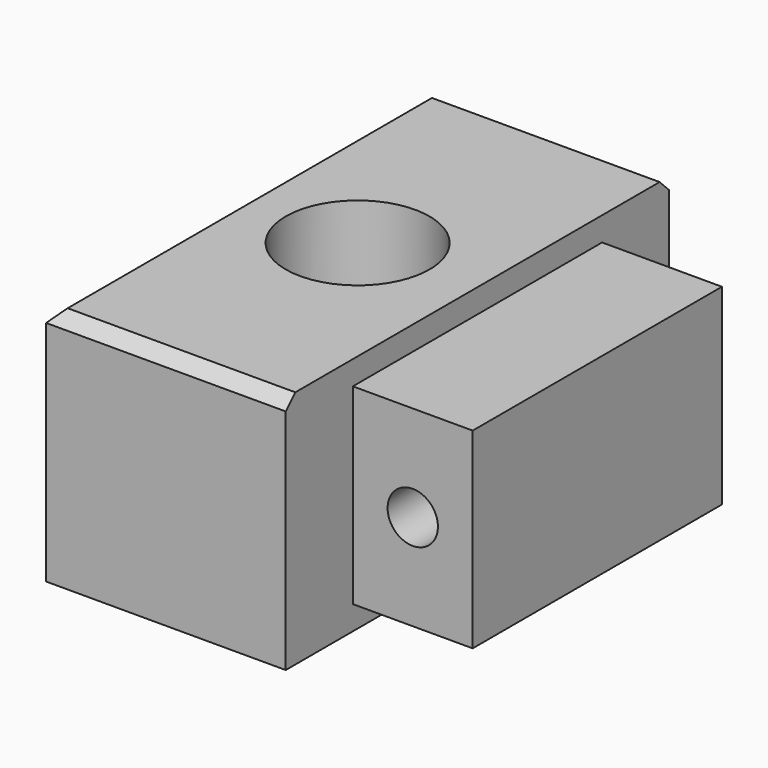
from build123d import *

# Parameters (mm, degrees)
F0_W      = 20
F0_H      = 40
F1_DEPTH  = 20
F3_D      = 12
F5_D      = 4.2
F5_DEPTH  = 5
F5_TIP    = 1.2618073
F8_SIZE   = 1
F9_W      = 26
F9_H      = 16
F10_DEPTH = 10
F12_D     = 4.2


# Not quite as in the source:
# - a feature of the source that left no trace in its solid (it failed there, or was rolled back) is left out


with BuildPart() as f1:
    # F0 (on Top) → F1 (new body)
    with BuildSketch(Plane.XY):
        with Locations((10, 20)):
            Rectangle(F0_W, F0_H)
    extrude(amount=F1_DEPTH)

    # F3 (through all)
    with Locations(Plane.XY.offset(20)):
        with Locations((10, 20)):
            Hole(F3_D / 2)

    # F5
    with Locations(Plane(origin=(0, 0, 0), x_dir=(0, -1, 0), z_dir=(-1, 0, 0))):
        with Locations((-20, 10)):
            Hole(F5_D / 2, depth=F5_DEPTH)
            with Locations((0, 0, -(F5_DEPTH + F5_TIP / 2))):  # 118° drill point
                Cone(0, F5_D / 2, F5_TIP, mode=Mode.SUBTRACT)

    # F8
    f8_edges = [f1.edges().sort_by_distance(p)[0] for p in [
        (10, 0, 20),
        (0, 20, 20),
        (10, 40, 20),
    ]]
    chamfer(f8_edges, length=F8_SIZE)

    # F9 (on face) → F10 (join)
    with BuildSketch(Plane.YZ.offset(20)):
        with Locations((20, 10)):
            Rectangle(F9_W, F9_H)
    extrude(amount=F10_DEPTH)

    # F12 (through all)
    with Locations(Plane.XZ.offset(-7)):
        with Locations((25, 10)):
            Hole(F12_D / 2)


solid = f1.part
